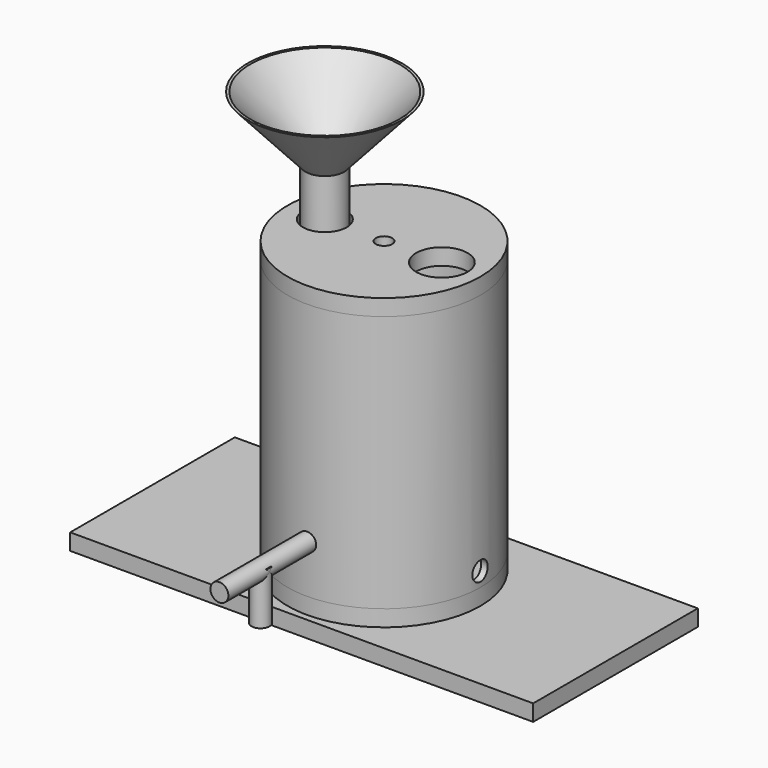
from build123d import *

# Parameters (mm, degrees)
F0_R       = 37.5
F0_R_2     = 2.25
F0_W       = 40.2
F0_H       = 40.2
F1_DEPTH   = 6.35
F3_R       = 37.5
F3_R_2     = 35
F4_DEPTH   = 100
F6_R       = 37.5
F6_R_2     = 8.5
F6_R_3     = 3.175
F6_R_4     = 10
F7_DEPTH   = 6.35
F9_W       = 180
F9_H       = 80
F9_W_2     = 42
F9_H_2     = 42
F10_DEPTH  = 6.35
F13_R      = 3.75
F14_DEPTH  = 75
F15_R      = 3.5
F16_DEPTH  = 80
F17_R      = 3.5
F18_DEPTH  = 20
F21_R      = 7.5
F22_DEPTH  = 25
F22_FACE_R = 7.5
F23_R      = 30
F25_R      = 6.5
F26_DEPTH  = 25
F27_R      = 29
F29_R      = 6.5


# Not quite as in the source:
# - a feature of the source that left no trace in its solid (it failed there, or was rolled back) is left out


with BuildPart() as f1:
    # F0 (on Top) → F1 (new body)
    with BuildSketch(Plane.XY):
        Circle(F0_R)
        with Locations((-20.1, 23)):
            Circle(F0_R_2, mode=Mode.SUBTRACT)
        Rectangle(F0_W, F0_H, mode=Mode.SUBTRACT)
        with Locations((20.1, 23)):
            Circle(F0_R_2, mode=Mode.SUBTRACT)
    extrude(amount=F1_DEPTH)


with BuildPart() as f4:
    # F3 (on offset) → F4 (new body)
    with BuildSketch(Plane.XY.offset(6.35)):
        Circle(F3_R)
        Circle(F3_R_2, mode=Mode.SUBTRACT)
    extrude(amount=F4_DEPTH)

    # F13 (on Right) → F14 (cut)
    with BuildSketch(Plane.YZ):
        with Locations((0, 12)):
            Circle(F13_R)
    extrude(amount=F14_DEPTH, mode=Mode.SUBTRACT)


with BuildPart() as f7:
    # F6 (on offset) → F7 (new body)
    with BuildSketch(Plane.XY.offset(106.35)):
        Circle(F6_R)
        with Locations((-23, 0)):
            Circle(F6_R_2, mode=Mode.SUBTRACT)
        Circle(F6_R_3, mode=Mode.SUBTRACT)
        with Locations((22.5, 0)):
            Circle(F6_R_4, mode=Mode.SUBTRACT)
    extrude(amount=F7_DEPTH)


with BuildPart() as f10:
    # F9 (on Top) → F10 (new body)
    with BuildSketch(Plane.XY):
        Rectangle(F9_W, F9_H)
        Rectangle(F9_W_2, F9_H_2, mode=Mode.SUBTRACT)
    extrude(amount=-F10_DEPTH)


with BuildPart() as f16:
    # F15 (on Front) → F16 (new body)
    with BuildSketch(Plane.XZ):
        with Locations((0, 25)):
            Circle(F15_R)
    extrude(amount=F16_DEPTH)

    # F17 (on offset) → F18 (join)
    with BuildSketch(Plane.XY.offset(6.35)):
        with Locations((0, -60)):
            Circle(F17_R)
    extrude(amount=F18_DEPTH)


with BuildPart() as f22:
    # F21 (on offset) → F22 (new body)
    with BuildSketch(Plane.XY.offset(106.35)):
        with Locations((-23, 0)):
            Circle(F21_R)
    extrude(amount=F22_DEPTH)

    # F22_face (on face) → F24 section 0
    with BuildSketch(Plane(origin=(-23, 0, 131.35), x_dir=(1, 0, 0), z_dir=(0, 0, 1))):
        Circle(F22_FACE_R)
    # F23 (on offset) → F24 section 1
    with BuildSketch(Plane.XY.offset(156.35)):
        with Locations((-23, 0)):
            Circle(F23_R)
    loft()

    # F25 (on offset) → F26 (cut)
    with BuildSketch(Plane.XY.offset(106.35)):
        with Locations((-23, 0)):
            Circle(F25_R)
    extrude(amount=F26_DEPTH, mode=Mode.SUBTRACT)

    # F27 (on offset) → F30 section 0
    with BuildSketch(Plane.XY.offset(156.35)):
        with Locations((-23, 0)):
            Circle(F27_R)
    # F29 (on offset) → F30 section 1
    with BuildSketch(Plane.XY.offset(131.35)):
        with Locations((-23, 0)):
            Circle(F29_R)
    loft(mode=Mode.SUBTRACT)


solid = Compound([f1.part, f4.part, f7.part, f10.part, f16.part, f22.part])
